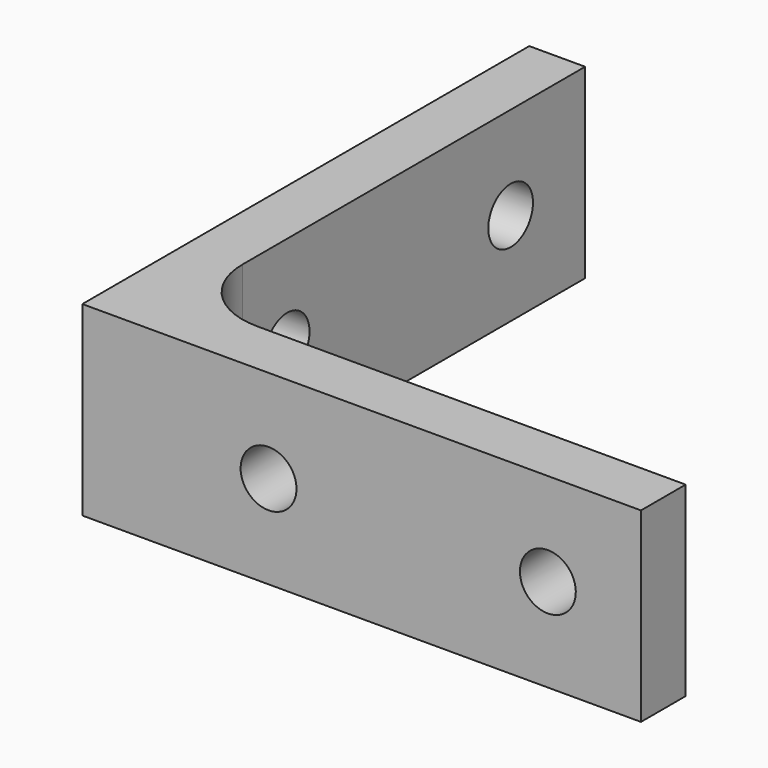
from build123d import *

# Parameters (mm, degrees)
F1_DEPTH   = 5
F4_D       = 3
F4_ON_F3_D = 3
F5_ANGLE   = 90


with BuildPart() as f1:
    # F0 (on Right) → F1 (new body, symmetric)
    with BuildSketch(Plane.YZ):
        with BuildLine():
            Line((3, 30), (0, 30))
            Line((0, 30), (0, 0))
            Line((0, 0), (30, 0))
            Line((30, 0), (30, 3))
            Line((30, 3), (7, 3))
            ThreePointArc((7, 3), (4.1715728753, 4.1715728753), (3, 7))
            Line((3, 7), (3, 30))
        make_face()
    extrude(amount=F1_DEPTH, both=True)

    # F4 (through all)
    with Locations(Plane.XY.offset(3)):
        with Locations((0, 25), (0, 10)):
            Hole(F4_D / 2)

    # F4 on F3 (through all)
    with Locations(Plane(origin=(0, 3, 0), x_dir=(-1, 0, 0), z_dir=(0, 1, 0))):
        with Locations((0, 25), (0, 10)):
            Hole(F4_ON_F3_D / 2)


with BuildPart() as f1_1:
    # F5: moved
    add(f1.part.rotate(Axis((5, 15, 0), (0, 1, 0)), F5_ANGLE))


solid = f1_1.part
